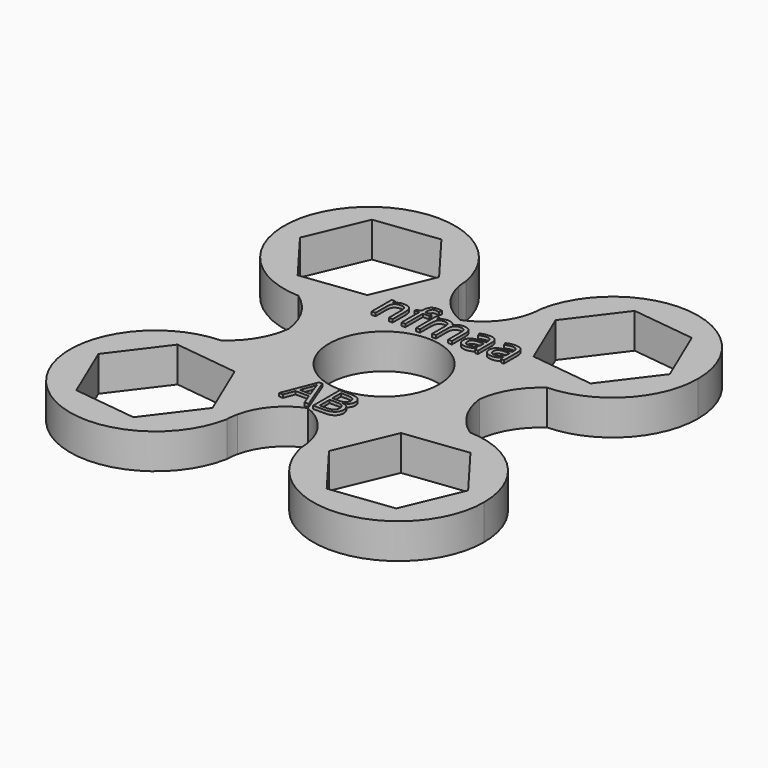
from build123d import *

# Parameters (mm, degrees)
F0_R           = 11.0128114896
F2_DEPTH       = 7.0104
F1_TEXT_SIZE   = 9.3311071396
F1_TEXT_SIZE_2 = 9.3311084331
F3_DEPTH       = 7.62


# Not quite as in the source:
# - Text() gives the source's letters only with a copy of the font that has no kerning and outlines rounded to 1/6400 em; it was checked with that copy


with BuildPart() as f2:
    # F0 (on Top) → F2 (new body)
    with BuildSketch(Plane.XY):
        with BuildLine():
            ThreePointArc((12.7990712305, -14.0870288637), (17.404987568, -7.7024031527), (19.0331449469, 0))
            ThreePointArc((19.0331449469, 0), (17.4049875909, 7.702403101), (12.7990713142, 14.0870287876))
            ThreePointArc((12.7990713142, 14.0870287876), (6.8607632879, 17.7536062161), (0, 19.0331449469))
            ThreePointArc((0, 19.0331449469), (-6.8607633047, 17.7536062096), (-12.799071341, 14.0870287633))
            ThreePointArc((-12.799071341, 14.0870287633), (-17.4049875982, 7.7024030845), (-19.0331449469, 0))
            ThreePointArc((-19.0331449469, 0), (-17.4049875412, -7.7024032133), (-12.7990711324, -14.0870289528))
            ThreePointArc((-12.7990711324, -14.0870289528), (-6.8607631733, -17.7536062604), (0, -19.0331449469))
            ThreePointArc((0, -19.0331449469), (6.8607632351, -17.7536062365), (12.7990712305, -14.0870288637))
        make_face()
        Circle(F0_R, mode=Mode.SUBTRACT)
        with BuildLine():
            ThreePointArc((24.8599982549, -9.661063392), (20.9119707268, -5.4545279665), (19.0331449469, 0))
            ThreePointArc((19.0331449469, 0), (17.404987568, -7.7024031527), (12.7990712305, -14.0870288637))
            ThreePointArc((12.7990712305, -14.0870288637), (18.3972516187, -10.6960579024), (24.8599982549, -9.661063392))
        make_face()
        with BuildLine():
            ThreePointArc((12.7990713142, 14.0870287876), (17.4049875909, 7.702403101), (19.0331449469, 0))
            ThreePointArc((19.0331449469, 0), (20.9119707268, 5.4545279665), (24.8599982549, 9.661063392))
            ThreePointArc((24.8599982549, 9.661063392), (18.3972516718, 10.6960578829), (12.7990713142, 14.0870287876))
        make_face()
        with BuildLine():
            ThreePointArc((0, 19.0331449469), (6.8607632879, 17.7536062161), (12.7990713142, 14.0870287876))
            ThreePointArc((12.7990713142, 14.0870287876), (8.5033122396, 20.1985496387), (7.2286770658, 27.559224765))
            ThreePointArc((7.2286770658, 27.559224765), (4.6745538054, 22.3973011968), (0, 19.0331449469))
        make_face()
        with BuildLine():
            ThreePointArc((7.2286770658, 27.559224765), (8.5033122396, 20.1985496387), (12.7990713142, 14.0870287876))
            ThreePointArc((12.7990713142, 14.0870287876), (18.3972516718, 10.6960578829), (24.8599982549, 9.661063392))
            ThreePointArc((24.8599982549, 9.661063392), (36.5520871531, 14.8583600371), (41.3476082867, 26.7208982259))
            ThreePointArc((41.3476082867, 26.7208982259), (25.8642568486, 43.7167848305), (7.5029518806, 29.8799928214))
            ThreePointArc((7.5029518806, 29.8799928214), (7.4227701569, 28.7128776123), (7.2286770658, 27.559224765))
        make_face()
        Polygon((16.607265395, 16.5507892681), (11.6349817483, 28.2787592779), (19.3055598882, 38.4488682357), (31.9484216749, 36.8910071837), (36.9207053216, 25.1630371739), (29.2501271817, 14.9929282161), align=None, mode=Mode.SUBTRACT)
        with BuildLine():
            ThreePointArc((7.2286770658, -27.559224765), (8.503312218, -20.198549691), (12.7990712305, -14.0870288637))
            ThreePointArc((12.7990712305, -14.0870288637), (6.8607632351, -17.7536062365), (0, -19.0331449469))
            ThreePointArc((0, -19.0331449469), (4.6745538054, -22.3973011968), (7.2286770658, -27.559224765))
        make_face()
        with BuildLine():
            ThreePointArc((24.8599982549, -9.661063392), (18.3972516187, -10.6960579024), (12.7990712305, -14.0870288637))
            ThreePointArc((12.7990712305, -14.0870288637), (8.503312218, -20.198549691), (7.2286770658, -27.559224765))
            ThreePointArc((7.2286770658, -27.559224765), (7.4227701569, -28.7128776123), (7.5029518806, -29.8799928214))
            ThreePointArc((7.5029518806, -29.8799928214), (25.8642568486, -43.7167848305), (41.3476082867, -26.7208982259))
            ThreePointArc((41.3476082867, -26.7208982259), (36.5520871531, -14.8583600371), (24.8599982549, -9.661063392))
        make_face()
        Polygon((19.3055598882, -38.4488682357), (11.6349817483, -28.2787592779), (16.607265395, -16.5507892681), (29.2501271817, -14.9929282161), (36.9207053216, -25.1630371739), (31.9484216749, -36.8910071837), align=None, mode=Mode.SUBTRACT)
        with BuildLine():
            ThreePointArc((-12.799071341, 14.0870287633), (-6.8607633047, 17.7536062096), (0, 19.0331449469))
            ThreePointArc((0, 19.0331449469), (-4.6745538054, 22.3973011968), (-7.2286770658, 27.559224765))
            ThreePointArc((-7.2286770658, 27.559224765), (-7.2132291309, 27.140188005), (-7.2080787832, 26.7208982259))
            ThreePointArc((-7.2080787832, 26.7208982259), (-8.6682822075, 19.8130429984), (-12.799071341, 14.0870287633))
        make_face()
        with BuildLine():
            ThreePointArc((-7.2286770658, -27.559224765), (-4.6745538054, -22.3973011968), (0, -19.0331449469))
            ThreePointArc((0, -19.0331449469), (-6.8607631733, -17.7536062604), (-12.7990711324, -14.0870289528))
            ThreePointArc((-12.7990711324, -14.0870289528), (-8.6682821505, -19.8130431272), (-7.2080787832, -26.7208982259))
            ThreePointArc((-7.2080787832, -26.7208982259), (-7.2132291309, -27.140188005), (-7.2286770658, -27.559224765))
        make_face()
        with BuildLine():
            ThreePointArc((-19.0331449469, 0), (-17.4049875982, 7.7024030845), (-12.799071341, 14.0870287633))
            ThreePointArc((-12.799071341, 14.0870287633), (-18.3972516888, 10.6960578767), (-24.8599982549, 9.661063392))
            ThreePointArc((-24.8599982549, 9.661063392), (-20.9119707268, 5.4545279665), (-19.0331449469, 0))
        make_face()
        with BuildLine():
            ThreePointArc((-24.8599982549, 9.661063392), (-18.3972516888, 10.6960578767), (-12.799071341, 14.0870287633))
            ThreePointArc((-12.799071341, 14.0870287633), (-8.6682822075, 19.8130429984), (-7.2080787832, 26.7208982259))
            ThreePointArc((-7.2080787832, 26.7208982259), (-7.2132291309, 27.140188005), (-7.2286770658, 27.559224765))
            ThreePointArc((-7.2286770658, 27.559224765), (-7.4227701569, 28.7128776123), (-7.5029518806, 29.8799928214))
            ThreePointArc((-7.5029518806, 29.8799928214), (-37.229772317, 37.8395496506), (-24.8599982549, 9.661063392))
        make_face()
        Polygon((-19.3055598882, 38.4488682357), (-11.6349817483, 28.2787592779), (-16.607265395, 16.5507892681), (-29.2501271817, 14.9929282161), (-36.9207053216, 25.1630371739), (-31.9484216749, 36.8910071837), align=None, mode=Mode.SUBTRACT)
        with BuildLine():
            ThreePointArc((-24.8599982549, -9.661063392), (-18.3972515565, -10.6960579252), (-12.7990711324, -14.0870289528))
            ThreePointArc((-12.7990711324, -14.0870289528), (-17.4049875412, -7.7024032133), (-19.0331449469, 0))
            ThreePointArc((-19.0331449469, 0), (-20.9119707268, -5.4545279665), (-24.8599982549, -9.661063392))
        make_face()
        with BuildLine():
            ThreePointArc((-7.2080787832, -26.7208982259), (-8.6682821505, -19.8130431272), (-12.7990711324, -14.0870289528))
            ThreePointArc((-12.7990711324, -14.0870289528), (-18.3972515565, -10.6960579252), (-24.8599982549, -9.661063392))
            ThreePointArc((-24.8599982549, -9.661063392), (-37.229772317, -37.8395496506), (-7.5029518806, -29.8799928214))
            ThreePointArc((-7.5029518806, -29.8799928214), (-7.4227701569, -28.7128776123), (-7.2286770658, -27.559224765))
            ThreePointArc((-7.2286770658, -27.559224765), (-7.2132291309, -27.140188005), (-7.2080787832, -26.7208982259))
        make_face()
        Polygon((-31.9484216749, -36.8910071837), (-36.9207053216, -25.1630371739), (-29.2501271817, -14.9929282161), (-16.607265395, -16.5507892681), (-11.6349817483, -28.2787592779), (-19.3055598882, -38.4488682357), align=None, mode=Mode.SUBTRACT)
    extrude(amount=F2_DEPTH)

    # F1 (on Top) → F3 (join)
    with BuildSketch(Plane.XY):
        with Locations((-12.6733398065, 11.7571949959)):
            Text('nfmaa', F1_TEXT_SIZE, font='Open Sans', text_align=(TextAlign.LEFT, TextAlign.BOTTOM))
        with Locations((-5.9549445286, -18.7809746712)):
            Text('AB', F1_TEXT_SIZE_2, font='Open Sans', text_align=(TextAlign.LEFT, TextAlign.BOTTOM))
    extrude(amount=F3_DEPTH)


solid = f2.part
